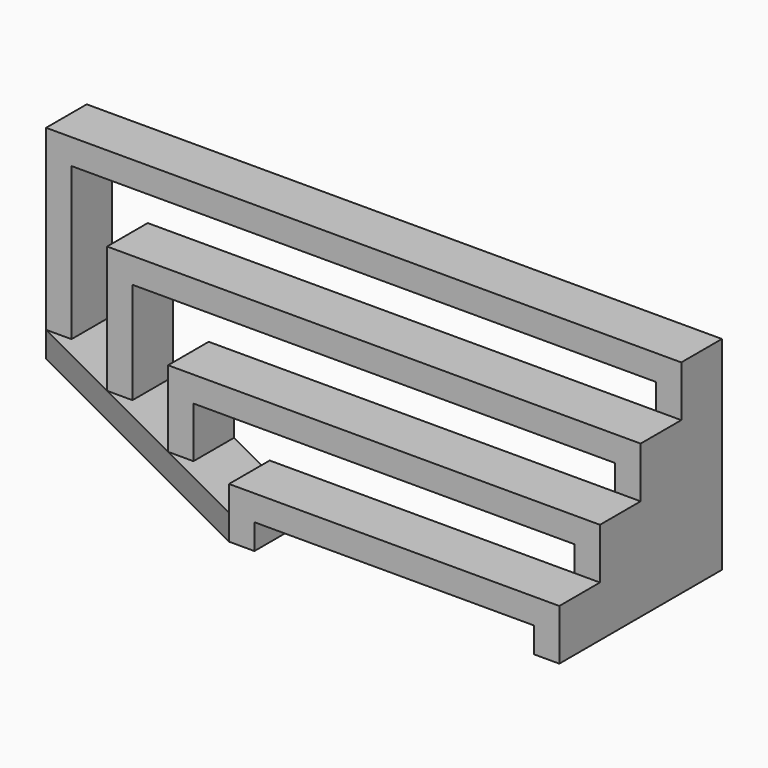
from build123d import *

# Parameters (mm, degrees)
F1_DEPTH  = 6.35
F3_DEPTH  = 12.7
F5_DEPTH  = 12.7
F7_DEPTH  = 12.7
F9_DEPTH  = 6.35
F11_DEPTH = 6.35


# Not quite as in the source:
# - ends of sketch curves that miss each other by under 0.0002 mm in the source are joined


with BuildPart() as f1:
    # F0 (on Front) → F1 (new body, symmetric)
    with BuildSketch(Plane.XZ):
        Polygon((0, -6.35), (0, 0), (-76.2, 0), (-76.2, -12.7), (-69.85, -12.7), (-69.85, -6.35), align=None)
    extrude(amount=F1_DEPTH, both=True)



with BuildPart() as f3:
    # F2 (on face) → F3 (new body)
    with BuildSketch(Plane(origin=(0, 6.35, 0), x_dir=(-1, 0, 0), z_dir=(0, 1, 0))):
        Polygon((101.6, 12.7), (0, 12.7), (0, 6.35), (95.25, 6.35), (95.25, -12.7), (101.6, -12.7), align=None)
    extrude(amount=F3_DEPTH)


with BuildPart() as f5:
    # F4 (on face) → F5 (new body)
    with BuildSketch(Plane(origin=(0, 19.05, 0), x_dir=(-1, 0, 0), z_dir=(0, 1, 0))):
        Polygon((127, 25.4), (0, 25.4), (0, 19.05), (120.65, 19.05), (120.65, -12.7), (127, -12.7), align=None)
    extrude(amount=F5_DEPTH)


with BuildPart() as f7:
    # F6 (on face) → F7 (new body)
    with BuildSketch(Plane(origin=(0, 31.75, 0), x_dir=(-1, 0, 0), z_dir=(0, 1, 0))):
        Polygon((152.4, 38.1), (0, 38.1), (0, 31.75), (146.05, 31.75), (146.05, -12.7), (152.4, -12.7), align=None)
    extrude(amount=F7_DEPTH)


with BuildPart() as f1_1:
    add(f1.part)

    add(f3.part)  # F9 merges F3

    add(f5.part)  # F9 merges F5

    add(f7.part)  # F9 merges F7
    # F8 (on Right) → F9 (join)
    with BuildSketch(Plane.YZ):
        Polygon((-6.35, -12.7), (44.45, -12.7), (44.45, 38.1), (31.75, 38.1), (31.75, 25.4), (19.05, 25.4), (19.05, 12.7), (6.35, 12.7), (6.35, 0), (-6.35, 0), align=None)
    extrude(amount=F9_DEPTH)

    # F10 (on face) → F11 (join)
    with BuildSketch(Plane(origin=(0, 0, -12.7), x_dir=(1, 0, 0), z_dir=(0, 0, -1))):
        Polygon((-152.4, -31.75), (-152.4, -44.45), (-146.05, -44.45), (-69.8499977589, -6.35), (-69.85, 6.35), (-76.2, 6.35), align=None)
    extrude(amount=-F11_DEPTH)


solid = f1_1.part
